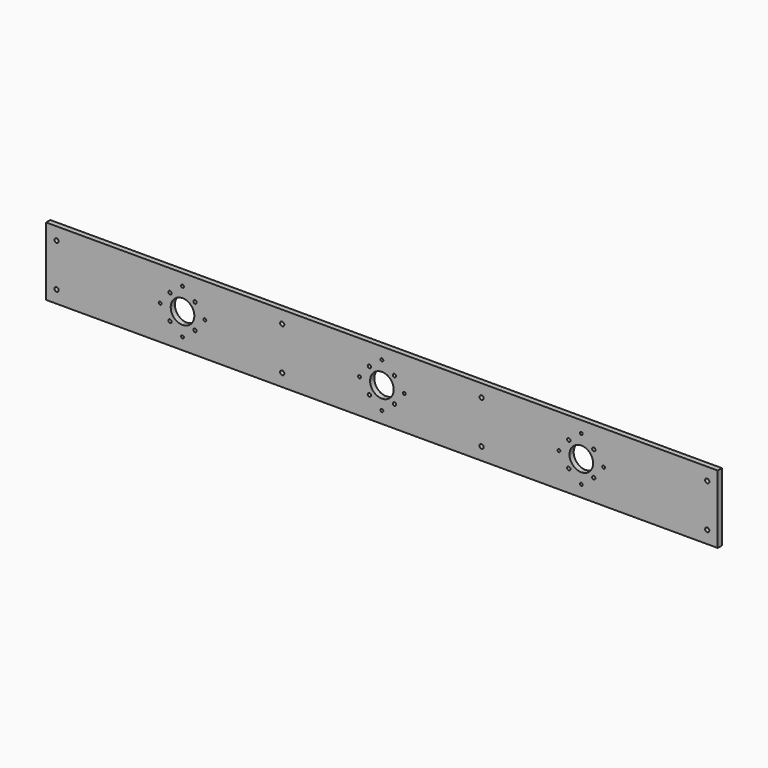
from build123d import *

# Parameters (mm, degrees)
F0_W     = 812.8
F0_H     = 82.55
F1_DEPTH = 6.35
F2_R     = 1.7272
F3_DEPTH = 6.35
F5_DEPTH = 6.35


# Not quite as in the source:
# - a pattern or mirror of a feature is missing from the dataset's text; its kind, count and spacing are read off the source's solid


with BuildPart() as f1:
    # F0 (on Front) → F1 (new body)
    with BuildSketch(Plane.XZ):
        Rectangle(F0_W, F0_H)
    extrude(amount=F1_DEPTH)

    # F2 (on face) → F3 (cut, through all)
    with BuildSketch(Plane.XZ.offset(6.35)):
        with BuildLine():
            Line((-227.0125, 0), (-241.3, 0))
            Line((-241.3, 0), (-241.3, -14.2875))
            ThreePointArc((-241.3, -14.2875), (-231.1972118638, -10.1027881362), (-227.0125, 0))
        make_face()
        with BuildLine():
            Line((-241.3, 14.2875), (-241.3, 0))
            Line((-241.3, 0), (-227.0125, 0))
            ThreePointArc((-227.0125, 0), (-231.1972118638, 10.1027881362), (-241.3, 14.2875))
        make_face()
        with BuildLine():
            ThreePointArc((-241.3, 14.2875), (-251.4027881362, 10.1027881362), (-255.5875, 0))
            Line((-255.5875, 0), (-241.3, 0))
            Line((-241.3, 0), (-241.3, 14.2875))
        make_face()
        with BuildLine():
            Line((-241.3, 0), (-255.5875, 0))
            ThreePointArc((-255.5875, 0), (-251.4027881362, -10.1027881362), (-241.3, -14.2875))
            Line((-241.3, -14.2875), (-241.3, 0))
        make_face()
        with BuildLine():
            Line((-256.45745, -15.15745), (-256.45745, -13.13815))
            ThreePointArc((-256.45745, -13.13815), (-257.8853107233, -16.5853107232), (-254.43815, -15.15745))
            Line((-254.43815, -15.15745), (-256.45745, -15.15745))
        make_face()
        with BuildLine():
            ThreePointArc((-254.43815, -15.15745), (-255.0295892767, -13.7295892768), (-256.45745, -13.13815))
            Line((-256.45745, -13.13815), (-256.45745, -15.15745))
            Line((-256.45745, -15.15745), (-254.43815, -15.15745))
        make_face()
        with BuildLine():
            ThreePointArc((-239.5728, -27.051), (-240.0786851675, -25.8296851675), (-241.3, -25.3238))
            ThreePointArc((-241.3, -25.3238), (-242.5213148325, -28.2723148325), (-239.5728, -27.051))
        make_face()
        with BuildLine():
            Line((-226.14255, -15.15745), (-228.16185, -15.15745))
            ThreePointArc((-228.16185, -15.15745), (-226.14255, -17.17675), (-224.12325, -15.15745))
            ThreePointArc((-224.12325, -15.15745), (-224.7146892767, -13.7295892768), (-226.14255, -13.13815))
            Line((-226.14255, -13.13815), (-226.14255, -15.15745))
        make_face()
        with BuildLine():
            ThreePointArc((-226.14255, -13.13815), (-227.5704107232, -13.7295892767), (-228.16185, -15.15745))
            Line((-228.16185, -15.15745), (-226.14255, -15.15745))
            Line((-226.14255, -15.15745), (-226.14255, -13.13815))
        make_face()
        with BuildLine():
            ThreePointArc((-224.12325, 15.15745), (-226.14255, 17.17675), (-228.16185, 15.15745))
            Line((-228.16185, 15.15745), (-226.14255, 15.15745))
            Line((-226.14255, 15.15745), (-226.14255, 13.13815))
            ThreePointArc((-226.14255, 13.13815), (-224.7146892767, 13.7295892768), (-224.12325, 15.15745))
        make_face()
        with BuildLine():
            Line((-226.14255, 15.15745), (-228.16185, 15.15745))
            ThreePointArc((-228.16185, 15.15745), (-227.5704107232, 13.7295892767), (-226.14255, 13.13815))
            Line((-226.14255, 13.13815), (-226.14255, 15.15745))
        make_face()
        with BuildLine():
            ThreePointArc((-212.5218, 0), (-214.249, 1.7272), (-215.9762, 0))
            ThreePointArc((-215.9762, 0), (-214.249, -1.7272), (-212.5218, 0))
        make_face()
        with BuildLine():
            ThreePointArc((-239.5728, 27.051), (-242.5213148325, 28.2723148325), (-241.3, 25.3238))
            ThreePointArc((-241.3, 25.3238), (-240.0786851675, 25.8296851675), (-239.5728, 27.051))
        make_face()
        with BuildLine():
            Line((-256.45745, 15.15745), (-256.45745, 13.13815))
            ThreePointArc((-256.45745, 13.13815), (-255.0295892767, 13.7295892768), (-254.43815, 15.15745))
            Line((-254.43815, 15.15745), (-256.45745, 15.15745))
        make_face()
        with BuildLine():
            ThreePointArc((-254.43815, 15.15745), (-257.8853107233, 16.5853107232), (-256.45745, 13.13815))
            Line((-256.45745, 13.13815), (-256.45745, 15.15745))
            Line((-256.45745, 15.15745), (-254.43815, 15.15745))
        make_face()
        with BuildLine():
            ThreePointArc((-270.0782, 0), (-268.351, -1.7272), (-266.6238, 0))
            Line((-266.6238, 0), (-270.0782, 0))
        make_face()
        with BuildLine():
            Line((-270.0782, 0), (-266.6238, 0))
            ThreePointArc((-266.6238, 0), (-268.351, 1.7272), (-270.0782, 0))
        make_face()
        with BuildLine():
            Line((14.2875, 0), (0, 0))
            Line((0, 0), (0, -14.2875))
            ThreePointArc((0, -14.2875), (10.1027881362, -10.1027881362), (14.2875, 0))
        make_face()
        with BuildLine():
            Line((0, -14.2875), (0, 0))
            Line((0, 0), (-14.2875, 0))
            ThreePointArc((-14.2875, 0), (-10.1027881362, -10.1027881362), (0, -14.2875))
        make_face()
        with BuildLine():
            Line((-14.2875, 0), (0, 0))
            Line((0, 0), (0, 14.2875))
            ThreePointArc((0, 14.2875), (-10.1027881362, 10.1027881362), (-14.2875, 0))
        make_face()
        with BuildLine():
            Line((0, 14.2875), (0, 0))
            Line((0, 0), (14.2875, 0))
            ThreePointArc((14.2875, 0), (10.1027881362, 10.1027881362), (0, 14.2875))
        make_face()
        with BuildLine():
            Line((15.15745, 15.15745), (15.15745, 13.13815))
            ThreePointArc((15.15745, 13.13815), (16.5853107233, 13.7295892768), (17.17675, 15.15745))
            ThreePointArc((17.17675, 15.15745), (15.15745, 17.17675), (13.13815, 15.15745))
            Line((13.13815, 15.15745), (15.15745, 15.15745))
        make_face()
        with BuildLine():
            ThreePointArc((13.13815, 15.15745), (13.7295892768, 13.7295892767), (15.15745, 13.13815))
            Line((15.15745, 13.13815), (15.15745, 15.15745))
            Line((15.15745, 15.15745), (13.13815, 15.15745))
        make_face()
        with BuildLine():
            ThreePointArc((1.7272, 27.051), (-1.2213148325, 28.2723148325), (0, 25.3238))
            ThreePointArc((0, 25.3238), (1.2213148325, 25.8296851675), (1.7272, 27.051))
        make_face()
        with BuildLine():
            Line((-15.15745, 15.15745), (-13.13815, 15.15745))
            ThreePointArc((-13.13815, 15.15745), (-16.5853107233, 16.5853107232), (-15.15745, 13.13815))
            Line((-15.15745, 13.13815), (-15.15745, 15.15745))
        make_face()
        with BuildLine():
            ThreePointArc((-15.15745, 13.13815), (-13.7295892767, 13.7295892768), (-13.13815, 15.15745))
            Line((-13.13815, 15.15745), (-15.15745, 15.15745))
            Line((-15.15745, 15.15745), (-15.15745, 13.13815))
        make_face()
        with BuildLine():
            ThreePointArc((-15.15745, -13.13815), (-16.5853107233, -16.5853107232), (-13.13815, -15.15745))
            Line((-13.13815, -15.15745), (-15.15745, -15.15745))
            Line((-15.15745, -15.15745), (-15.15745, -13.13815))
        make_face()
        with BuildLine():
            Line((-15.15745, -15.15745), (-13.13815, -15.15745))
            ThreePointArc((-13.13815, -15.15745), (-13.7295892767, -13.7295892768), (-15.15745, -13.13815))
            Line((-15.15745, -13.13815), (-15.15745, -15.15745))
        make_face()
        with BuildLine():
            ThreePointArc((1.7272, -27.051), (1.2213148325, -25.8296851675), (0, -25.3238))
            ThreePointArc((0, -25.3238), (-1.2213148325, -28.2723148325), (1.7272, -27.051))
        make_face()
        with BuildLine():
            ThreePointArc((17.17675, -15.15745), (16.5853107233, -13.7295892768), (15.15745, -13.13815))
            Line((15.15745, -13.13815), (15.15745, -15.15745))
            Line((15.15745, -15.15745), (13.13815, -15.15745))
            ThreePointArc((13.13815, -15.15745), (15.15745, -17.17675), (17.17675, -15.15745))
        make_face()
        with BuildLine():
            Line((15.15745, -15.15745), (15.15745, -13.13815))
            ThreePointArc((15.15745, -13.13815), (13.7295892768, -13.7295892767), (13.13815, -15.15745))
            Line((13.13815, -15.15745), (15.15745, -15.15745))
        make_face()
        with Locations((-27.051, 0.1607450395)):
            Circle(F2_R)
        with BuildLine():
            ThreePointArc((28.7782, 0), (27.051, 1.7272), (25.3238, 0))
            ThreePointArc((25.3238, 0), (27.051, -1.7272), (28.7782, 0))
        make_face()
        with BuildLine():
            ThreePointArc((241.3, -14.2875), (251.4027881362, -10.1027881362), (255.5875, 0))
            Line((255.5875, 0), (241.3, 0))
            Line((241.3, 0), (241.3, -14.2875))
        make_face()
        with BuildLine():
            Line((241.3, 0), (255.5875, 0))
            ThreePointArc((255.5875, 0), (251.4027881362, 10.1027881362), (241.3, 14.2875))
            Line((241.3, 14.2875), (241.3, 0))
        make_face()
        with BuildLine():
            Line((227.0125, 0), (241.3, 0))
            Line((241.3, 0), (241.3, 14.2875))
            ThreePointArc((241.3, 14.2875), (231.1972118638, 10.1027881362), (227.0125, 0))
        make_face()
        with BuildLine():
            Line((241.3, -14.2875), (241.3, 0))
            Line((241.3, 0), (227.0125, 0))
            ThreePointArc((227.0125, 0), (231.1972118638, -10.1027881362), (241.3, -14.2875))
        make_face()
        with BuildLine():
            ThreePointArc((258.47675, -15.15745), (257.8853107232, -13.7295892768), (256.45745, -13.13815))
            Line((256.45745, -13.13815), (256.45745, -15.15745))
            Line((256.45745, -15.15745), (254.43815, -15.15745))
            ThreePointArc((254.43815, -15.15745), (256.45745, -17.17675), (258.47675, -15.15745))
        make_face()
        with BuildLine():
            Line((256.45745, -15.15745), (256.45745, -13.13815))
            ThreePointArc((256.45745, -13.13815), (255.0295892767, -13.7295892768), (254.43815, -15.15745))
            Line((254.43815, -15.15745), (256.45745, -15.15745))
        make_face()
        with BuildLine():
            ThreePointArc((243.0272, -27.051), (242.5213148325, -25.8296851675), (241.3, -25.3238))
            ThreePointArc((241.3, -25.3238), (240.0786851675, -28.2723148325), (243.0272, -27.051))
        make_face()
        with BuildLine():
            ThreePointArc((266.6238, 0), (268.351, -1.7272), (270.0782, 0))
            Line((270.0782, 0), (266.6238, 0))
        make_face()
        with BuildLine():
            Line((266.6238, 0), (270.0782, 0))
            ThreePointArc((270.0782, 0), (268.351, 1.7272), (266.6238, 0))
        make_face()
        with BuildLine():
            Line((256.45745, 15.15745), (256.45745, 13.13815))
            ThreePointArc((256.45745, 13.13815), (257.8853107232, 13.7295892768), (258.47675, 15.15745))
            ThreePointArc((258.47675, 15.15745), (256.45745, 17.17675), (254.43815, 15.15745))
            Line((254.43815, 15.15745), (256.45745, 15.15745))
        make_face()
        with BuildLine():
            ThreePointArc((254.43815, 15.15745), (255.0295892767, 13.7295892768), (256.45745, 13.13815))
            Line((256.45745, 13.13815), (256.45745, 15.15745))
            Line((256.45745, 15.15745), (254.43815, 15.15745))
        make_face()
        with BuildLine():
            ThreePointArc((243.0272, 27.051), (240.0786851675, 28.2723148325), (241.3, 25.3238))
            ThreePointArc((241.3, 25.3238), (242.5213148325, 25.8296851675), (243.0272, 27.051))
        make_face()
        with BuildLine():
            ThreePointArc((226.14255, 13.13815), (227.5704107233, 13.7295892768), (228.16185, 15.15745))
            Line((228.16185, 15.15745), (226.14255, 15.15745))
            Line((226.14255, 15.15745), (226.14255, 13.13815))
        make_face()
        with BuildLine():
            Line((226.14255, 15.15745), (228.16185, 15.15745))
            ThreePointArc((228.16185, 15.15745), (224.7146892767, 16.5853107232), (226.14255, 13.13815))
            Line((226.14255, 13.13815), (226.14255, 15.15745))
        make_face()
        with BuildLine():
            ThreePointArc((226.14255, -13.13815), (224.7146892767, -16.5853107232), (228.16185, -15.15745))
            Line((228.16185, -15.15745), (226.14255, -15.15745))
            Line((226.14255, -15.15745), (226.14255, -13.13815))
        make_face()
        with BuildLine():
            Line((226.14255, -15.15745), (228.16185, -15.15745))
            ThreePointArc((228.16185, -15.15745), (227.5704107233, -13.7295892768), (226.14255, -13.13815))
            Line((226.14255, -13.13815), (226.14255, -15.15745))
        make_face()
        with Locations((214.249, 0)):
            Circle(F2_R)
    extrude(amount=-F3_DEPTH, mode=Mode.SUBTRACT)

    # F4 (on face) → F5 (cut, through all)
    with BuildSketch(Plane.XZ.offset(6.35)):
        with BuildLine():
            ThreePointArc((-391.16, 26.035), (-391.9039487758, 27.8310512242), (-393.7, 28.575))
            Line((-393.7, 28.575), (-393.7, 23.495))
            ThreePointArc((-393.7, 23.495), (-391.9039487758, 24.2389487758), (-391.16, 26.035))
        make_face()
        with BuildLine():
            ThreePointArc((-391.16, -26.035), (-391.9039487758, -24.2389487758), (-393.7, -23.495))
            Line((-393.7, -23.495), (-393.7, -28.575))
            ThreePointArc((-393.7, -28.575), (-391.9039487758, -27.8310512242), (-391.16, -26.035))
        make_face()
        with BuildLine():
            Line((-393.7, -28.575), (-393.7, -23.495))
            ThreePointArc((-393.7, -23.495), (-396.24, -26.035), (-393.7, -28.575))
        make_face()
        with BuildLine():
            Line((-393.7, 23.495), (-393.7, 28.575))
            ThreePointArc((-393.7, 28.575), (-396.24, 26.035), (-393.7, 23.495))
        make_face()
        with BuildLine():
            ThreePointArc((-118.11, 26.035), (-118.8539487758, 27.8310512242), (-120.65, 28.575))
            Line((-120.65, 28.575), (-120.65, 23.495))
            ThreePointArc((-120.65, 23.495), (-118.8539487758, 24.2389487758), (-118.11, 26.035))
        make_face()
        with BuildLine():
            ThreePointArc((-118.11, -26.035), (-118.8539487758, -24.2389487758), (-120.65, -23.495))
            Line((-120.65, -23.495), (-120.65, -28.575))
            ThreePointArc((-120.65, -28.575), (-118.8539487758, -27.8310512242), (-118.11, -26.035))
        make_face()
        with BuildLine():
            Line((-120.65, -28.575), (-120.65, -23.495))
            ThreePointArc((-120.65, -23.495), (-123.19, -26.035), (-120.65, -28.575))
        make_face()
        with BuildLine():
            Line((-120.65, 23.495), (-120.65, 28.575))
            ThreePointArc((-120.65, 28.575), (-123.19, 26.035), (-120.65, 23.495))
        make_face()
    f5 = extrude(amount=-F5_DEPTH, mode=Mode.SUBTRACT)

    # F5_copies: F5 across plane
    add(f5.mirror(Plane(origin=(0, 0, 0), x_dir=(0, 0, 1), z_dir=(1, 0, 0))), mode=Mode.SUBTRACT)


solid = f1.part
